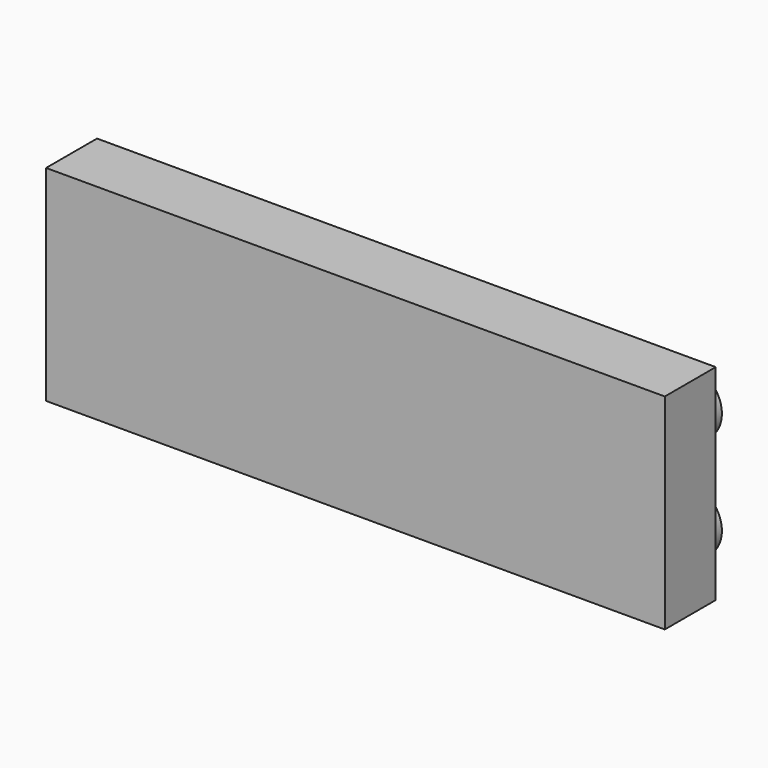
from build123d import *

# Parameters (mm, degrees)
F0_R     = 2.46
F1_DEPTH = 4.92
F2_R     = 2.46
F4_DEPTH = 1.4


# Not quite as in the source:
# - the program builds the solid bodies; features that only make, move or delete a surface that nothing else refers to are left out


with BuildPart() as f1:
    # F0 (on Front) → F1 (new body)
    with BuildSketch(Plane.XZ):
        Polygon((-47.81, 0), (0, 0), (0, 15.85), (-47.81, 15.85), (-47.81, 4.5985402539), align=None)
        with BuildLine():
            ThreePointArc((-42.89, 4.5985402539), (-45.35, 2.1385402539), (-47.81, 4.5985402539))
            ThreePointArc((-47.81, 4.5985402539), (-45.3923948453, 7.0581749173), (-42.8914612381, 4.6833173524))
            ThreePointArc((-42.8914612381, 4.6833173524), (-42.8903653367, 4.6409350993), (-42.89, 4.5985402539))
        make_face(mode=Mode.SUBTRACT)
        with BuildLine():
            ThreePointArc((-37.9729224851, 4.7680947078), (-40.3905275113, 2.3084600467), (-42.8914612381, 4.6833173524))
            ThreePointArc((-42.8914612381, 4.6833173524), (-40.475317459, 7.227729369), (-37.9729224851, 4.7680947078))
        make_face(mode=Mode.SUBTRACT)
        with Locations((-26.7290156335, 5.1733576693)):
            Circle(F0_R, mode=Mode.SUBTRACT)
        with Locations((-20.1186146587, 3.1614964828)):
            Circle(F0_R, mode=Mode.SUBTRACT)
        with Locations((-13.7956207618, 3.1614964828)):
            Circle(F0_R, mode=Mode.SUBTRACT)
        with BuildLine():
            ThreePointArc((-6.4156207618, 3.1614964828), (-8.8756207618, 0.7014964828), (-11.3356207618, 3.1614964828))
            ThreePointArc((-11.3356207618, 3.1614964828), (-8.8756207618, 5.6214964828), (-6.4156207618, 3.1614964828))
        make_face(mode=Mode.SUBTRACT)
        with Locations((-43.3987230062, 10.9215332195)):
            Circle(F0_R, mode=Mode.SUBTRACT)
        with Locations((-34.7764603794, 10.9215332195)):
            Circle(F0_R, mode=Mode.SUBTRACT)
        with BuildLine():
            ThreePointArc((-24.2718000183, 10.8045228756), (-29.1883194387, 10.9800549535), (-24.2690156335, 10.9215332195))
            ThreePointArc((-24.2690156335, 10.9215332195), (-24.2697118282, 10.8630114856), (-24.2718000183, 10.8045228756))
        make_face(mode=Mode.SUBTRACT)
        with BuildLine():
            ThreePointArc((-19.3545844044, 10.6875125042), (-21.8731061521, 8.2282086993), (-24.2718000183, 10.8045228756))
            ThreePointArc((-24.2718000183, 10.8045228756), (-21.7560626567, 13.1468163092), (-19.3545844044, 10.6875125042))
        make_face(mode=Mode.SUBTRACT)
        with Locations((-13.2208028808, 10.9215332195)):
            Circle(F0_R, mode=Mode.SUBTRACT)
        with Locations((-6.3229943626, 10.9215332195)):
            Circle(F0_R, mode=Mode.SUBTRACT)
        with BuildLine():
            ThreePointArc((-42.8914612381, 4.6833173524), (-45.3923948453, 7.0581749173), (-47.81, 4.5985402539))
            ThreePointArc((-47.81, 4.5985402539), (-45.35, 2.1385402539), (-42.89, 4.5985402539))
            ThreePointArc((-42.89, 4.5985402539), (-42.8903653367, 4.6409350993), (-42.8914612381, 4.6833173524))
        make_face()
        with BuildLine():
            ThreePointArc((-37.9729224851, 4.7680947078), (-40.475317459, 7.227729369), (-42.8914612381, 4.6833173524))
            ThreePointArc((-42.8914612381, 4.6833173524), (-40.3905275113, 2.3084600467), (-37.9729224851, 4.7680947078))
        make_face()
        with Locations((-43.3987230062, 10.9215332195)):
            Circle(F0_R)
        with Locations((-26.7290156335, 5.1733576693)):
            Circle(F0_R)
        with BuildLine():
            ThreePointArc((-24.2718000183, 10.8045228756), (-24.2697118282, 10.8630114856), (-24.2690156335, 10.9215332195))
            ThreePointArc((-24.2690156335, 10.9215332195), (-29.1883194387, 10.9800549535), (-24.2718000183, 10.8045228756))
        make_face()
        with BuildLine():
            ThreePointArc((-19.3545844044, 10.6875125042), (-21.7560626567, 13.1468163092), (-24.2718000183, 10.8045228756))
            ThreePointArc((-24.2718000183, 10.8045228756), (-21.8731061521, 8.2282086993), (-19.3545844044, 10.6875125042))
        make_face()
        with Locations((-20.1186146587, 3.1614964828)):
            Circle(F0_R)
        with Locations((-13.7956207618, 3.1614964828)):
            Circle(F0_R)
        with BuildLine():
            ThreePointArc((-6.4156207618, 3.1614964828), (-8.8756207618, 5.6214964828), (-11.3356207618, 3.1614964828))
            ThreePointArc((-11.3356207618, 3.1614964828), (-8.8756207618, 0.7014964828), (-6.4156207618, 3.1614964828))
        make_face()
        with Locations((-13.2208028808, 10.9215332195)):
            Circle(F0_R)
        with Locations((-6.3229943626, 10.9215332195)):
            Circle(F0_R)
        with Locations((-34.7764603794, 10.9215332195)):
            Circle(F0_R)
    extrude(amount=F1_DEPTH)

    # F2 (on Front) → F4 (join)
    with BuildSketch(Plane.XZ):
        with Locations((-42.9514177962, 11.845)):
            Circle(F2_R)
        with Locations((-42.9514177962, 3.875)):
            Circle(F2_R)
        with Locations((-34.9824780926, 11.975)):
            Circle(F2_R)
        with Locations((-34.9824780926, 4.005)):
            Circle(F2_R)
        with Locations((-27.0125882826, 11.9330903837)):
            Circle(F2_R)
        with Locations((-19.0425920932, 11.9408840209)):
            Circle(F2_R)
        with Locations((-11.0725940906, 3.9652414555)):
            Circle(F2_R)
        with Locations((-11.0725940906, 11.9352414555)):
            Circle(F2_R)
        with Locations((-3.1026442768, 3.9369577962)):
            Circle(F2_R)
        with Locations((-3.1026442768, 11.9069577962)):
            Circle(F2_R)
        with Locations((-19.0425920932, 3.9708840209)):
            Circle(F2_R)
        with Locations((-27.0125882826, 3.9630903837)):
            Circle(F2_R)
    extrude(amount=-F4_DEPTH)


solid = f1.part
